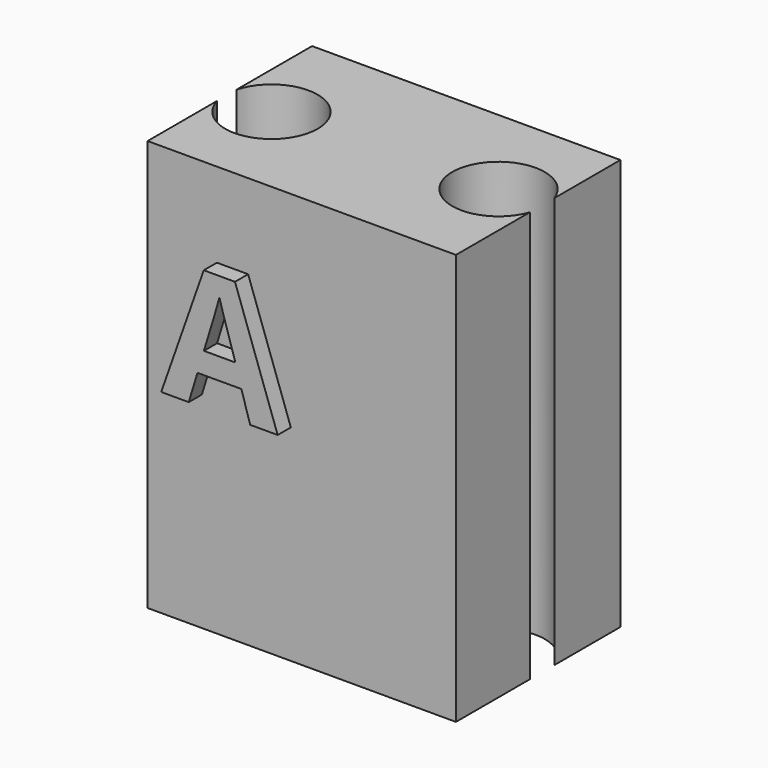
from build123d import *

# Parameters (mm, degrees)
F0_W         = 4.7625
F0_H         = 6.35
F1_DEPTH     = 3.175
F4_D         = 1.428242
F6_D         = 1.428242
F7_TEXT_SIZE = 2.6068626151
F8_DEPTH     = 0.254


# Not quite as in the source:
# - the program builds the solid bodies; features that only make, move or delete a surface that nothing else refers to are left out
# - Text() gives the source's letters only with a copy of the font that has no kerning and outlines rounded to 1/6400 em; it was checked with that copy


with BuildPart() as f1:
    # F0 (on Front) → F1 (new body)
    with BuildSketch(Plane.XZ):
        Rectangle(F0_W, F0_H)
    extrude(amount=F1_DEPTH)

    # F4 (through all)
    with Locations(Plane.XY.offset(3.175)):
        with Locations((-1.6927157994, -1.6449075192)):
            Hole(F4_D / 2)

    # F6 (through all)
    with Locations(Plane.XY.offset(3.175)):
        with Locations((1.7077114899, -1.5113163972)):
            Hole(F6_D / 2)

    # F7 (on face) → F8 (join)
    with BuildSketch(Plane.XZ.offset(3.175)):
        with Locations((-1.9677739521, 0)):
            Text('A', F7_TEXT_SIZE, font='Open Sans', font_style=FontStyle.BOLD, text_align=(TextAlign.LEFT, TextAlign.BOTTOM))
    extrude(amount=F8_DEPTH)


solid = f1.part
